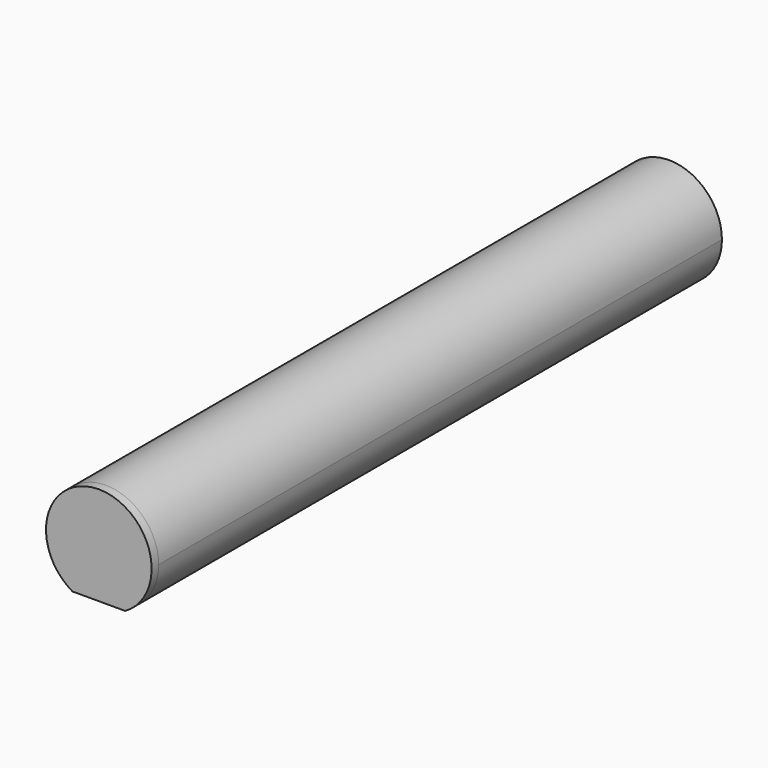
from build123d import *

# Parameters (mm, degrees)
F1_DEPTH  = 127
F2_W      = 8.6666238164
F2_H      = 1.5875
F2_W_2    = 1.2
F3_DEPTH  = 127
F4_OFFSET = 0.5
F6_DEPTH  = 1.5875
F7_R      = 2.5
F8_DEPTH  = 1.5875


with BuildPart() as f1:
    # F0 (on Front) → F1 (new body)
    with BuildSketch(Plane.XZ):
        with BuildLine():
            ThreePointArc((-7.9201799173, -0.5240766425), (-0.262181384, 7.9331687976), (7.9375, 0))
            ThreePointArc((7.9375, 0), (7.9331687976, -0.262181384), (7.9201799173, -0.5240766425))
            ThreePointArc((7.9201799173, -0.5240766425), (7.3187167756, -3.0725056564), (5.9208119082, -5.2865766425))
            ThreePointArc((5.9208119082, -5.2865766425), (5.0080832408, -6.1581660016), (3.96875, -6.8740766425))
            Line((3.96875, -6.8740766425), (4.7625, -8.248891971))
            ThreePointArc((4.7625, -8.248891971), (8.248891971, -4.7625), (9.525, 0))
            ThreePointArc((9.525, 0), (-4.7625, 8.248891971), (-4.7625, -8.248891971))
            Line((-4.7625, -8.248891971), (-3.96875, -6.8740766425))
            ThreePointArc((-3.96875, -6.8740766425), (-5.0080832408, -6.1581660016), (-5.9208119082, -5.2865766425))
            ThreePointArc((-5.9208119082, -5.2865766425), (-7.3187167756, -3.0725056564), (-7.9201799173, -0.5240766425))
        make_face()
        with BuildLine():
            Line((-4.3333119082, -0.5240766425), (-7.9201799173, -0.5240766425))
            ThreePointArc((-7.9201799173, -0.5240766425), (-7.3187167756, -3.0725056564), (-5.9208119082, -5.2865766425))
            Line((-5.9208119082, -5.2865766425), (-4.3333119082, -5.2865766425))
            Line((-4.3333119082, -5.2865766425), (-4.3333119082, -0.5240766425))
        make_face()
        with BuildLine():
            ThreePointArc((5.9208119082, -5.2865766425), (7.3187167756, -3.0725056564), (7.9201799173, -0.5240766425))
            Line((7.9201799173, -0.5240766425), (4.3333119082, -0.5240766425))
            Line((4.3333119082, -0.5240766425), (4.3333119082, -5.2865766425))
            Line((4.3333119082, -5.2865766425), (5.9208119082, -5.2865766425))
        make_face()
    extrude(amount=F1_DEPTH)


with BuildPart() as f3:
    # F2 (on face) → F3 (new body, through all)
    with BuildSketch(Plane(origin=(0, 0, 0), x_dir=(-1, 0, 0), z_dir=(0, 1, 0))):
        with Locations((0, -2.9053266425)):
            Rectangle(F2_W, F2_H)
        with Locations((-4.9333119082, -2.9053266425)):
            Rectangle(F2_W_2, F2_H)
        with Locations((4.9333119082, -2.9053266425)):
            Rectangle(F2_W_2, F2_H)
    extrude(amount=-F3_DEPTH)


with BuildPart() as f1_1:
    add(f1.part)

    # F4: cut F3, made larger all round first
    f4_tool = offset(f3.part, amount=F4_OFFSET, kind=Kind.INTERSECTION, mode=Mode.PRIVATE)
    add(f4_tool, mode=Mode.SUBTRACT)

    # F5 (on face) → F6 (join)
    with BuildSketch(Plane.XZ.offset(127)):
        with BuildLine():
            Line((-4.7625, -8.248891971), (4.7625, -8.248891971))
            ThreePointArc((4.7625, -8.248891971), (0, 9.525), (-4.7625, -8.248891971))
        make_face()
    extrude(amount=F6_DEPTH)


with BuildPart() as f3_1:
    add(f3.part)

    # F7 (on face) → F8 (cut, through all)
    with BuildSketch(Plane(origin=(0, 0, -3.6990766425), x_dir=(1, 0, 0), z_dir=(0, 0, -1))):
        with Locations((0, 12.7)):
            Circle(F7_R)
        with Locations((0, 38.1)):
            Circle(F7_R)
        with Locations((0, 63.5)):
            Circle(F7_R)
        with Locations((0, 88.9)):
            Circle(F7_R)
        with Locations((0, 114.3)):
            Circle(F7_R)
    extrude(amount=-F8_DEPTH, mode=Mode.SUBTRACT)


solid = Compound([f1_1.part, f3_1.part])
